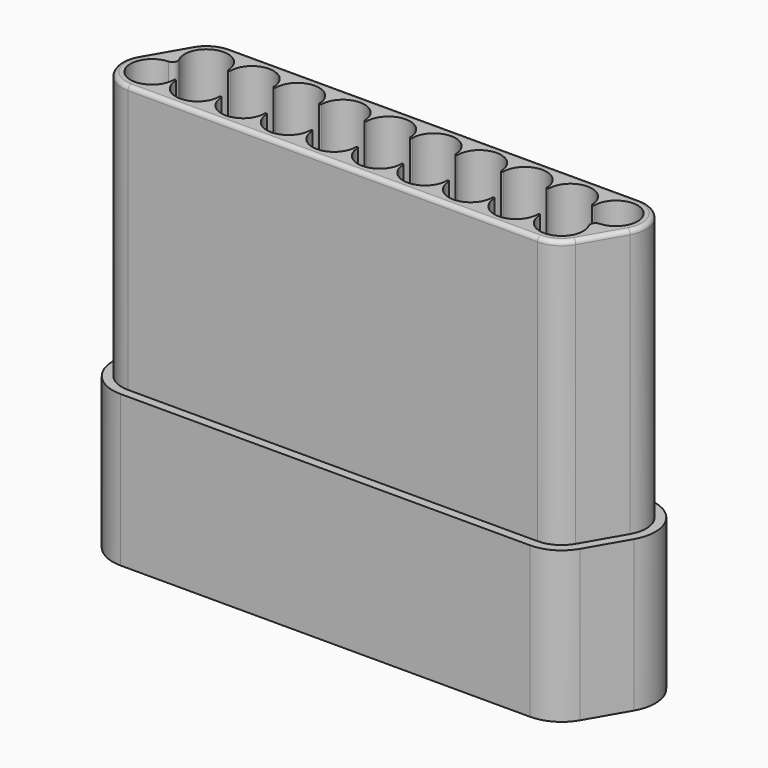
from build123d import *

# Parameters (mm, degrees)
F1_DEPTH = 75
F2_DEPTH = 25
F3_DEPTH = 3.2
F4_R     = 0.8


# Not quite as in the source:
# - a feature names something its author has since deleted; it is built from what else it names


with BuildPart() as f1:
    # F0 (on Top) → F1 (new body)
    with BuildSketch(Plane.XY):
        with BuildLine():
            Line((-0.6430435314, 10.1862159322), (-4.8930435314, 2.825))
            ThreePointArc((-4.8930435314, 2.825), (-4.8930435314, -2.825), (0, -5.65))
            Line((0, -5.65), (76.5, -5.65))
            ThreePointArc((76.5, -5.65), (79.325, -4.8930435314), (81.3930435314, -2.825))
            Line((81.3930435314, -2.825), (85.6430435314, 4.5362159322))
            ThreePointArc((85.6430435314, 4.5362159322), (85.6430435314, 10.1862159322), (80.75, 13.0112159322))
            Line((80.75, 13.0112159322), (4.25, 13.0112159322))
            ThreePointArc((4.25, 13.0112159322), (1.425, 12.2542594635), (-0.6430435314, 10.1862159322))
        make_face()
        with BuildLine():
            ThreePointArc((4.45, 0), (4.25, -0.2), (4.05, 0))
            ThreePointArc((4.05, 0), (-2.7957165477, -2.9302677326), (-0.1902315974, 4.0455298713))
            ThreePointArc((-0.1902315974, 4.0455298713), (0.6288230416, 4.5444261358), (0.651352561, 5.5031963925))
            ThreePointArc((0.651352561, 5.5031963925), (3.2939723142, 11.2967605024), (8.3, 7.3612159322))
            ThreePointArc((8.3, 7.3612159322), (8.5, 7.5612159322), (8.7, 7.3612159322))
            ThreePointArc((8.7, 7.3612159322), (12.75, 11.4112159322), (16.8, 7.3612159322))
            ThreePointArc((16.8, 7.3612159322), (17, 7.5612159322), (17.2, 7.3612159322))
            ThreePointArc((17.2, 7.3612159322), (21.25, 11.4112159322), (25.3, 7.3612159322))
            ThreePointArc((25.3, 7.3612159322), (25.5, 7.5612159322), (25.7, 7.3612159322))
            ThreePointArc((25.7, 7.3612159322), (29.75, 11.4112159322), (33.8, 7.3612159322))
            ThreePointArc((33.8, 7.3612159322), (34, 7.5612159322), (34.2, 7.3612159322))
            ThreePointArc((34.2, 7.3612159322), (38.25, 11.4112159322), (42.3, 7.3612159322))
            ThreePointArc((42.3, 7.3612159322), (42.5, 7.5612159322), (42.7, 7.3612159322))
            ThreePointArc((42.7, 7.3612159322), (46.75, 11.4112159322), (50.8, 7.3612159322))
            ThreePointArc((50.8, 7.3612159322), (51, 7.5612159322), (51.2, 7.3612159322))
            ThreePointArc((51.2, 7.3612159322), (55.25, 11.4112159322), (59.3, 7.3612159322))
            ThreePointArc((59.3, 7.3612159322), (59.5, 7.5612159322), (59.7, 7.3612159322))
            ThreePointArc((59.7, 7.3612159322), (63.75, 11.4112159322), (67.8, 7.3612159322))
            ThreePointArc((67.8, 7.3612159322), (68, 7.5612159322), (68.2, 7.3612159322))
            ThreePointArc((68.2, 7.3612159322), (72.25, 11.4112159322), (76.3, 7.3612159322))
            ThreePointArc((76.3, 7.3612159322), (76.5, 7.5612159322), (76.7, 7.3612159322))
            ThreePointArc((76.7, 7.3612159322), (80.75, 11.4112159322), (84.8, 7.3612159322))
            ThreePointArc((84.8, 7.3612159322), (83.6802677326, 4.5654993844), (80.9402315974, 3.3156860609))
            ThreePointArc((80.9402315974, 3.3156860609), (80.1211769584, 2.8167897964), (80.098647439, 1.8580195397))
            ThreePointArc((80.098647439, 1.8580195397), (80.4355445702, 0.9560276858), (80.55, 0))
            ThreePointArc((80.55, 0), (76.5, -4.05), (72.45, 0))
            ThreePointArc((72.45, 0), (72.25, -0.2), (72.05, 0))
            ThreePointArc((72.05, 0), (68, -4.05), (63.95, 0))
            ThreePointArc((63.95, 0), (63.75, -0.2), (63.55, 0))
            ThreePointArc((63.55, 0), (59.5, -4.05), (55.45, 0))
            ThreePointArc((55.45, 0), (55.25, -0.2), (55.05, 0))
            ThreePointArc((55.05, 0), (51, -4.05), (46.95, 0))
            ThreePointArc((46.95, 0), (46.75, -0.2), (46.55, 0))
            ThreePointArc((46.55, 0), (42.5, -4.05), (38.45, 0))
            ThreePointArc((38.45, 0), (38.25, -0.2), (38.05, 0))
            ThreePointArc((38.05, 0), (34, -4.05), (29.95, 0))
            ThreePointArc((29.95, 0), (29.75, -0.2), (29.55, 0))
            ThreePointArc((29.55, 0), (25.5, -4.05), (21.45, 0))
            ThreePointArc((21.45, 0), (21.25, -0.2), (21.05, 0))
            ThreePointArc((21.05, 0), (17, -4.05), (12.95, 0))
            ThreePointArc((12.95, 0), (12.75, -0.2), (12.55, 0))
            ThreePointArc((12.55, 0), (8.5, -4.05), (4.45, 0))
        make_face(mode=Mode.SUBTRACT)
        with BuildLine():
            ThreePointArc((4.45, 0), (4.25, 0.2), (4.05, 0))
            ThreePointArc((4.05, 0), (4.25, -0.2), (4.45, 0))
        make_face()
        with BuildLine():
            ThreePointArc((8.7, 7.3612159322), (8.5, 7.5612159322), (8.3, 7.3612159322))
            ThreePointArc((8.3, 7.3612159322), (8.5, 7.1612159322), (8.7, 7.3612159322))
        make_face()
        with BuildLine():
            ThreePointArc((12.95, 0), (12.75, 0.2), (12.55, 0))
            ThreePointArc((12.55, 0), (12.75, -0.2), (12.95, 0))
        make_face()
        with BuildLine():
            ThreePointArc((17.2, 7.3612159322), (17, 7.5612159322), (16.8, 7.3612159322))
            ThreePointArc((16.8, 7.3612159322), (17, 7.1612159322), (17.2, 7.3612159322))
        make_face()
        with BuildLine():
            ThreePointArc((21.45, 0), (21.25, 0.2), (21.05, 0))
            ThreePointArc((21.05, 0), (21.25, -0.2), (21.45, 0))
        make_face()
        with BuildLine():
            ThreePointArc((25.7, 7.3612159322), (25.5, 7.5612159322), (25.3, 7.3612159322))
            ThreePointArc((25.3, 7.3612159322), (25.5, 7.1612159322), (25.7, 7.3612159322))
        make_face()
        with BuildLine():
            ThreePointArc((29.95, 0), (29.75, 0.2), (29.55, 0))
            ThreePointArc((29.55, 0), (29.75, -0.2), (29.95, 0))
        make_face()
        with BuildLine():
            ThreePointArc((34.2, 7.3612159322), (34, 7.5612159322), (33.8, 7.3612159322))
            ThreePointArc((33.8, 7.3612159322), (34, 7.1612159322), (34.2, 7.3612159322))
        make_face()
        with BuildLine():
            ThreePointArc((38.45, 0), (38.25, 0.2), (38.05, 0))
            ThreePointArc((38.05, 0), (38.25, -0.2), (38.45, 0))
        make_face()
        with BuildLine():
            ThreePointArc((42.7, 7.3612159322), (42.5, 7.5612159322), (42.3, 7.3612159322))
            ThreePointArc((42.3, 7.3612159322), (42.5, 7.1612159322), (42.7, 7.3612159322))
        make_face()
        with BuildLine():
            ThreePointArc((46.95, 0), (46.75, 0.2), (46.55, 0))
            ThreePointArc((46.55, 0), (46.75, -0.2), (46.95, 0))
        make_face()
        with BuildLine():
            ThreePointArc((51.2, 7.3612159322), (51, 7.5612159322), (50.8, 7.3612159322))
            ThreePointArc((50.8, 7.3612159322), (51, 7.1612159322), (51.2, 7.3612159322))
        make_face()
        with BuildLine():
            ThreePointArc((55.45, 0), (55.25, 0.2), (55.05, 0))
            ThreePointArc((55.05, 0), (55.25, -0.2), (55.45, 0))
        make_face()
        with BuildLine():
            ThreePointArc((59.7, 7.3612159322), (59.5, 7.5612159322), (59.3, 7.3612159322))
            ThreePointArc((59.3, 7.3612159322), (59.5, 7.1612159322), (59.7, 7.3612159322))
        make_face()
        with BuildLine():
            ThreePointArc((63.95, 0), (63.75, 0.2), (63.55, 0))
            ThreePointArc((63.55, 0), (63.75, -0.2), (63.95, 0))
        make_face()
        with BuildLine():
            ThreePointArc((68.2, 7.3612159322), (68, 7.5612159322), (67.8, 7.3612159322))
            ThreePointArc((67.8, 7.3612159322), (68, 7.1612159322), (68.2, 7.3612159322))
        make_face()
        with BuildLine():
            ThreePointArc((72.45, 0), (72.25, 0.2), (72.05, 0))
            ThreePointArc((72.05, 0), (72.25, -0.2), (72.45, 0))
        make_face()
        with BuildLine():
            ThreePointArc((76.7, 7.3612159322), (76.5, 7.5612159322), (76.3, 7.3612159322))
            ThreePointArc((76.3, 7.3612159322), (76.5, 7.1612159322), (76.7, 7.3612159322))
        make_face()
    extrude(amount=F1_DEPTH)

    # F0 (on Top) → F2 (join)
    with BuildSketch(Plane.XY):
        with BuildLine():
            Line((-2.1152867178, 11.0362159322), (-6.3652867178, 3.675))
            ThreePointArc((-6.3652867178, 3.675), (-6.3652867178, -3.675), (0, -7.35))
            Line((0, -7.35), (76.5, -7.35))
            ThreePointArc((76.5, -7.35), (80.175, -6.3652867178), (82.8652867178, -3.675))
            Line((82.8652867178, -3.675), (87.1152867178, 3.6862159322))
            ThreePointArc((87.1152867178, 3.6862159322), (87.1152867178, 11.0362159322), (80.75, 14.7112159322))
            Line((80.75, 14.7112159322), (4.25, 14.7112159322))
            ThreePointArc((4.25, 14.7112159322), (0.575, 13.72650265), (-2.1152867178, 11.0362159322))
        make_face()
        with BuildLine():
            ThreePointArc((0, -5.65), (-4.8930435314, -2.825), (-4.8930435314, 2.825))
            Line((-4.8930435314, 2.825), (-0.6430435314, 10.1862159322))
            ThreePointArc((-0.6430435314, 10.1862159322), (1.425, 12.2542594635), (4.25, 13.0112159322))
            Line((4.25, 13.0112159322), (80.75, 13.0112159322))
            ThreePointArc((80.75, 13.0112159322), (85.6430435314, 10.1862159322), (85.6430435314, 4.5362159322))
            Line((85.6430435314, 4.5362159322), (81.3930435314, -2.825))
            ThreePointArc((81.3930435314, -2.825), (79.325, -4.8930435314), (76.5, -5.65))
            Line((76.5, -5.65), (0, -5.65))
        make_face(mode=Mode.SUBTRACT)
    extrude(amount=F2_DEPTH)

    # F0 (on Top) → F3 (join)
    with BuildSketch(Plane.XY):
        with BuildLine():
            Line((-2.1152867178, 11.0362159322), (-6.3652867178, 3.675))
            ThreePointArc((-6.3652867178, 3.675), (-6.3652867178, -3.675), (0, -7.35))
            Line((0, -7.35), (76.5, -7.35))
            ThreePointArc((76.5, -7.35), (80.175, -6.3652867178), (82.8652867178, -3.675))
            Line((82.8652867178, -3.675), (87.1152867178, 3.6862159322))
            ThreePointArc((87.1152867178, 3.6862159322), (87.1152867178, 11.0362159322), (80.75, 14.7112159322))
            Line((80.75, 14.7112159322), (4.25, 14.7112159322))
            ThreePointArc((4.25, 14.7112159322), (0.575, 13.72650265), (-2.1152867178, 11.0362159322))
        make_face()
        with BuildLine():
            ThreePointArc((0, -5.65), (-4.8930435314, -2.825), (-4.8930435314, 2.825))
            Line((-4.8930435314, 2.825), (-0.6430435314, 10.1862159322))
            ThreePointArc((-0.6430435314, 10.1862159322), (1.425, 12.2542594635), (4.25, 13.0112159322))
            Line((4.25, 13.0112159322), (80.75, 13.0112159322))
            ThreePointArc((80.75, 13.0112159322), (85.6430435314, 10.1862159322), (85.6430435314, 4.5362159322))
            Line((85.6430435314, 4.5362159322), (81.3930435314, -2.825))
            ThreePointArc((81.3930435314, -2.825), (79.325, -4.8930435314), (76.5, -5.65))
            Line((76.5, -5.65), (0, -5.65))
        make_face(mode=Mode.SUBTRACT)
        with BuildLine():
            Line((-0.6430435314, 10.1862159322), (-4.8930435314, 2.825))
            ThreePointArc((-4.8930435314, 2.825), (-4.8930435314, -2.825), (0, -5.65))
            Line((0, -5.65), (76.5, -5.65))
            ThreePointArc((76.5, -5.65), (79.325, -4.8930435314), (81.3930435314, -2.825))
            Line((81.3930435314, -2.825), (85.6430435314, 4.5362159322))
            ThreePointArc((85.6430435314, 4.5362159322), (85.6430435314, 10.1862159322), (80.75, 13.0112159322))
            Line((80.75, 13.0112159322), (4.25, 13.0112159322))
            ThreePointArc((4.25, 13.0112159322), (1.425, 12.2542594635), (-0.6430435314, 10.1862159322))
        make_face()
        with BuildLine():
            ThreePointArc((4.45, 0), (4.25, -0.2), (4.05, 0))
            ThreePointArc((4.05, 0), (-2.7957165477, -2.9302677326), (-0.1902315974, 4.0455298713))
            ThreePointArc((-0.1902315974, 4.0455298713), (0.6288230416, 4.5444261358), (0.651352561, 5.5031963925))
            ThreePointArc((0.651352561, 5.5031963925), (3.2939723142, 11.2967605024), (8.3, 7.3612159322))
            ThreePointArc((8.3, 7.3612159322), (8.5, 7.5612159322), (8.7, 7.3612159322))
            ThreePointArc((8.7, 7.3612159322), (12.75, 11.4112159322), (16.8, 7.3612159322))
            ThreePointArc((16.8, 7.3612159322), (17, 7.5612159322), (17.2, 7.3612159322))
            ThreePointArc((17.2, 7.3612159322), (21.25, 11.4112159322), (25.3, 7.3612159322))
            ThreePointArc((25.3, 7.3612159322), (25.5, 7.5612159322), (25.7, 7.3612159322))
            ThreePointArc((25.7, 7.3612159322), (29.75, 11.4112159322), (33.8, 7.3612159322))
            ThreePointArc((33.8, 7.3612159322), (34, 7.5612159322), (34.2, 7.3612159322))
            ThreePointArc((34.2, 7.3612159322), (38.25, 11.4112159322), (42.3, 7.3612159322))
            ThreePointArc((42.3, 7.3612159322), (42.5, 7.5612159322), (42.7, 7.3612159322))
            ThreePointArc((42.7, 7.3612159322), (46.75, 11.4112159322), (50.8, 7.3612159322))
            ThreePointArc((50.8, 7.3612159322), (51, 7.5612159322), (51.2, 7.3612159322))
            ThreePointArc((51.2, 7.3612159322), (55.25, 11.4112159322), (59.3, 7.3612159322))
            ThreePointArc((59.3, 7.3612159322), (59.5, 7.5612159322), (59.7, 7.3612159322))
            ThreePointArc((59.7, 7.3612159322), (63.75, 11.4112159322), (67.8, 7.3612159322))
            ThreePointArc((67.8, 7.3612159322), (68, 7.5612159322), (68.2, 7.3612159322))
            ThreePointArc((68.2, 7.3612159322), (72.25, 11.4112159322), (76.3, 7.3612159322))
            ThreePointArc((76.3, 7.3612159322), (76.5, 7.5612159322), (76.7, 7.3612159322))
            ThreePointArc((76.7, 7.3612159322), (80.75, 11.4112159322), (84.8, 7.3612159322))
            ThreePointArc((84.8, 7.3612159322), (83.6802677326, 4.5654993844), (80.9402315974, 3.3156860609))
            ThreePointArc((80.9402315974, 3.3156860609), (80.1211769584, 2.8167897964), (80.098647439, 1.8580195397))
            ThreePointArc((80.098647439, 1.8580195397), (80.4355445702, 0.9560276858), (80.55, 0))
            ThreePointArc((80.55, 0), (76.5, -4.05), (72.45, 0))
            ThreePointArc((72.45, 0), (72.25, -0.2), (72.05, 0))
            ThreePointArc((72.05, 0), (68, -4.05), (63.95, 0))
            ThreePointArc((63.95, 0), (63.75, -0.2), (63.55, 0))
            ThreePointArc((63.55, 0), (59.5, -4.05), (55.45, 0))
            ThreePointArc((55.45, 0), (55.25, -0.2), (55.05, 0))
            ThreePointArc((55.05, 0), (51, -4.05), (46.95, 0))
            ThreePointArc((46.95, 0), (46.75, -0.2), (46.55, 0))
            ThreePointArc((46.55, 0), (42.5, -4.05), (38.45, 0))
            ThreePointArc((38.45, 0), (38.25, -0.2), (38.05, 0))
            ThreePointArc((38.05, 0), (34, -4.05), (29.95, 0))
            ThreePointArc((29.95, 0), (29.75, -0.2), (29.55, 0))
            ThreePointArc((29.55, 0), (25.5, -4.05), (21.45, 0))
            ThreePointArc((21.45, 0), (21.25, -0.2), (21.05, 0))
            ThreePointArc((21.05, 0), (17, -4.05), (12.95, 0))
            ThreePointArc((12.95, 0), (12.75, -0.2), (12.55, 0))
            ThreePointArc((12.55, 0), (8.5, -4.05), (4.45, 0))
        make_face(mode=Mode.SUBTRACT)
        with BuildLine():
            ThreePointArc((-0.1902315974, 4.0455298713), (2.7957165477, 2.9302677326), (4.05, 0))
            ThreePointArc((4.05, 0), (4.25, 0.2), (4.45, 0))
            ThreePointArc((4.45, 0), (8.5, 4.05), (12.55, 0))
            ThreePointArc((12.55, 0), (12.75, 0.2), (12.95, 0))
            ThreePointArc((12.95, 0), (17, 4.05), (21.05, 0))
            ThreePointArc((21.05, 0), (21.25, 0.2), (21.45, 0))
            ThreePointArc((21.45, 0), (25.5, 4.05), (29.55, 0))
            ThreePointArc((29.55, 0), (29.75, 0.2), (29.95, 0))
            ThreePointArc((29.95, 0), (34, 4.05), (38.05, 0))
            ThreePointArc((38.05, 0), (38.25, 0.2), (38.45, 0))
            ThreePointArc((38.45, 0), (42.5, 4.05), (46.55, 0))
            ThreePointArc((46.55, 0), (46.75, 0.2), (46.95, 0))
            ThreePointArc((46.95, 0), (51, 4.05), (55.05, 0))
            ThreePointArc((55.05, 0), (55.25, 0.2), (55.45, 0))
            ThreePointArc((55.45, 0), (59.5, 4.05), (63.55, 0))
            ThreePointArc((63.55, 0), (63.75, 0.2), (63.95, 0))
            ThreePointArc((63.95, 0), (68, 4.05), (72.05, 0))
            ThreePointArc((72.05, 0), (72.25, 0.2), (72.45, 0))
            ThreePointArc((72.45, 0), (75.5439723142, 3.9355445702), (80.098647439, 1.8580195397))
            ThreePointArc((80.098647439, 1.8580195397), (80.1211769584, 2.8167897964), (80.9402315974, 3.3156860609))
            ThreePointArc((80.9402315974, 3.3156860609), (77.9542834523, 4.4309481996), (76.7, 7.3612159322))
            ThreePointArc((76.7, 7.3612159322), (76.5, 7.1612159322), (76.3, 7.3612159322))
            ThreePointArc((76.3, 7.3612159322), (72.25, 3.3112159322), (68.2, 7.3612159322))
            ThreePointArc((68.2, 7.3612159322), (68, 7.1612159322), (67.8, 7.3612159322))
            ThreePointArc((67.8, 7.3612159322), (63.75, 3.3112159322), (59.7, 7.3612159322))
            ThreePointArc((59.7, 7.3612159322), (59.5, 7.1612159322), (59.3, 7.3612159322))
            ThreePointArc((59.3, 7.3612159322), (55.25, 3.3112159322), (51.2, 7.3612159322))
            ThreePointArc((51.2, 7.3612159322), (51, 7.1612159322), (50.8, 7.3612159322))
            ThreePointArc((50.8, 7.3612159322), (46.75, 3.3112159322), (42.7, 7.3612159322))
            ThreePointArc((42.7, 7.3612159322), (42.5, 7.1612159322), (42.3, 7.3612159322))
            ThreePointArc((42.3, 7.3612159322), (38.25, 3.3112159322), (34.2, 7.3612159322))
            ThreePointArc((34.2, 7.3612159322), (34, 7.1612159322), (33.8, 7.3612159322))
            ThreePointArc((33.8, 7.3612159322), (29.75, 3.3112159322), (25.7, 7.3612159322))
            ThreePointArc((25.7, 7.3612159322), (25.5, 7.1612159322), (25.3, 7.3612159322))
            ThreePointArc((25.3, 7.3612159322), (21.25, 3.3112159322), (17.2, 7.3612159322))
            ThreePointArc((17.2, 7.3612159322), (17, 7.1612159322), (16.8, 7.3612159322))
            ThreePointArc((16.8, 7.3612159322), (12.75, 3.3112159322), (8.7, 7.3612159322))
            ThreePointArc((8.7, 7.3612159322), (8.5, 7.1612159322), (8.3, 7.3612159322))
            ThreePointArc((8.3, 7.3612159322), (5.2060276858, 3.425671362), (0.651352561, 5.5031963925))
            ThreePointArc((0.651352561, 5.5031963925), (0.6288230416, 4.5444261358), (-0.1902315974, 4.0455298713))
        make_face()
        with BuildLine():
            ThreePointArc((-0.1902315974, 4.0455298713), (-2.7957165477, -2.9302677326), (4.05, 0))
            ThreePointArc((4.05, 0), (2.7957165477, 2.9302677326), (-0.1902315974, 4.0455298713))
        make_face()
        with BuildLine():
            ThreePointArc((12.55, 0), (8.5, 4.05), (4.45, 0))
            ThreePointArc((4.45, 0), (8.5, -4.05), (12.55, 0))
        make_face()
        with BuildLine():
            ThreePointArc((8.3, 7.3612159322), (3.2939723142, 11.2967605024), (0.651352561, 5.5031963925))
            ThreePointArc((0.651352561, 5.5031963925), (5.2060276858, 3.425671362), (8.3, 7.3612159322))
        make_face()
        with BuildLine():
            ThreePointArc((21.05, 0), (17, 4.05), (12.95, 0))
            ThreePointArc((12.95, 0), (17, -4.05), (21.05, 0))
        make_face()
        with BuildLine():
            ThreePointArc((16.8, 7.3612159322), (12.75, 11.4112159322), (8.7, 7.3612159322))
            ThreePointArc((8.7, 7.3612159322), (12.75, 3.3112159322), (16.8, 7.3612159322))
        make_face()
        with BuildLine():
            ThreePointArc((29.55, 0), (25.5, 4.05), (21.45, 0))
            ThreePointArc((21.45, 0), (25.5, -4.05), (29.55, 0))
        make_face()
        with BuildLine():
            ThreePointArc((25.3, 7.3612159322), (21.25, 11.4112159322), (17.2, 7.3612159322))
            ThreePointArc((17.2, 7.3612159322), (21.25, 3.3112159322), (25.3, 7.3612159322))
        make_face()
        with BuildLine():
            ThreePointArc((38.05, 0), (34, 4.05), (29.95, 0))
            ThreePointArc((29.95, 0), (34, -4.05), (38.05, 0))
        make_face()
        with BuildLine():
            ThreePointArc((33.8, 7.3612159322), (29.75, 11.4112159322), (25.7, 7.3612159322))
            ThreePointArc((25.7, 7.3612159322), (29.75, 3.3112159322), (33.8, 7.3612159322))
        make_face()
        with BuildLine():
            ThreePointArc((46.55, 0), (42.5, 4.05), (38.45, 0))
            ThreePointArc((38.45, 0), (42.5, -4.05), (46.55, 0))
        make_face()
        with BuildLine():
            ThreePointArc((42.3, 7.3612159322), (38.25, 11.4112159322), (34.2, 7.3612159322))
            ThreePointArc((34.2, 7.3612159322), (38.25, 3.3112159322), (42.3, 7.3612159322))
        make_face()
        with BuildLine():
            ThreePointArc((55.05, 0), (51, 4.05), (46.95, 0))
            ThreePointArc((46.95, 0), (51, -4.05), (55.05, 0))
        make_face()
        with BuildLine():
            ThreePointArc((50.8, 7.3612159322), (46.75, 11.4112159322), (42.7, 7.3612159322))
            ThreePointArc((42.7, 7.3612159322), (46.75, 3.3112159322), (50.8, 7.3612159322))
        make_face()
        with BuildLine():
            ThreePointArc((63.55, 0), (59.5, 4.05), (55.45, 0))
            ThreePointArc((55.45, 0), (59.5, -4.05), (63.55, 0))
        make_face()
        with BuildLine():
            ThreePointArc((59.3, 7.3612159322), (55.25, 11.4112159322), (51.2, 7.3612159322))
            ThreePointArc((51.2, 7.3612159322), (55.25, 3.3112159322), (59.3, 7.3612159322))
        make_face()
        with BuildLine():
            ThreePointArc((72.05, 0), (68, 4.05), (63.95, 0))
            ThreePointArc((63.95, 0), (68, -4.05), (72.05, 0))
        make_face()
        with BuildLine():
            ThreePointArc((67.8, 7.3612159322), (63.75, 11.4112159322), (59.7, 7.3612159322))
            ThreePointArc((59.7, 7.3612159322), (63.75, 3.3112159322), (67.8, 7.3612159322))
        make_face()
        with BuildLine():
            ThreePointArc((80.098647439, 1.8580195397), (75.5439723142, 3.9355445702), (72.45, 0))
            ThreePointArc((72.45, 0), (76.5, -4.05), (80.55, 0))
            ThreePointArc((80.55, 0), (80.4355445702, 0.9560276858), (80.098647439, 1.8580195397))
        make_face()
        with BuildLine():
            ThreePointArc((76.3, 7.3612159322), (72.25, 11.4112159322), (68.2, 7.3612159322))
            ThreePointArc((68.2, 7.3612159322), (72.25, 3.3112159322), (76.3, 7.3612159322))
        make_face()
        with BuildLine():
            ThreePointArc((76.7, 7.3612159322), (77.9542834523, 4.4309481996), (80.9402315974, 3.3156860609))
            ThreePointArc((80.9402315974, 3.3156860609), (83.6802677326, 4.5654993844), (84.8, 7.3612159322))
            ThreePointArc((84.8, 7.3612159322), (80.75, 11.4112159322), (76.7, 7.3612159322))
        make_face()
        with BuildLine():
            ThreePointArc((4.45, 0), (4.25, 0.2), (4.05, 0))
            ThreePointArc((4.05, 0), (4.25, -0.2), (4.45, 0))
        make_face()
        with BuildLine():
            ThreePointArc((12.95, 0), (12.75, 0.2), (12.55, 0))
            ThreePointArc((12.55, 0), (12.75, -0.2), (12.95, 0))
        make_face()
        with BuildLine():
            ThreePointArc((8.7, 7.3612159322), (8.5, 7.5612159322), (8.3, 7.3612159322))
            ThreePointArc((8.3, 7.3612159322), (8.5, 7.1612159322), (8.7, 7.3612159322))
        make_face()
        with BuildLine():
            ThreePointArc((21.45, 0), (21.25, 0.2), (21.05, 0))
            ThreePointArc((21.05, 0), (21.25, -0.2), (21.45, 0))
        make_face()
        with BuildLine():
            ThreePointArc((17.2, 7.3612159322), (17, 7.5612159322), (16.8, 7.3612159322))
            ThreePointArc((16.8, 7.3612159322), (17, 7.1612159322), (17.2, 7.3612159322))
        make_face()
        with BuildLine():
            ThreePointArc((29.95, 0), (29.75, 0.2), (29.55, 0))
            ThreePointArc((29.55, 0), (29.75, -0.2), (29.95, 0))
        make_face()
        with BuildLine():
            ThreePointArc((25.7, 7.3612159322), (25.5, 7.5612159322), (25.3, 7.3612159322))
            ThreePointArc((25.3, 7.3612159322), (25.5, 7.1612159322), (25.7, 7.3612159322))
        make_face()
        with BuildLine():
            ThreePointArc((38.45, 0), (38.25, 0.2), (38.05, 0))
            ThreePointArc((38.05, 0), (38.25, -0.2), (38.45, 0))
        make_face()
        with BuildLine():
            ThreePointArc((34.2, 7.3612159322), (34, 7.5612159322), (33.8, 7.3612159322))
            ThreePointArc((33.8, 7.3612159322), (34, 7.1612159322), (34.2, 7.3612159322))
        make_face()
        with BuildLine():
            ThreePointArc((46.95, 0), (46.75, 0.2), (46.55, 0))
            ThreePointArc((46.55, 0), (46.75, -0.2), (46.95, 0))
        make_face()
        with BuildLine():
            ThreePointArc((42.7, 7.3612159322), (42.5, 7.5612159322), (42.3, 7.3612159322))
            ThreePointArc((42.3, 7.3612159322), (42.5, 7.1612159322), (42.7, 7.3612159322))
        make_face()
        with BuildLine():
            ThreePointArc((55.45, 0), (55.25, 0.2), (55.05, 0))
            ThreePointArc((55.05, 0), (55.25, -0.2), (55.45, 0))
        make_face()
        with BuildLine():
            ThreePointArc((51.2, 7.3612159322), (51, 7.5612159322), (50.8, 7.3612159322))
            ThreePointArc((50.8, 7.3612159322), (51, 7.1612159322), (51.2, 7.3612159322))
        make_face()
        with BuildLine():
            ThreePointArc((63.95, 0), (63.75, 0.2), (63.55, 0))
            ThreePointArc((63.55, 0), (63.75, -0.2), (63.95, 0))
        make_face()
        with BuildLine():
            ThreePointArc((59.7, 7.3612159322), (59.5, 7.5612159322), (59.3, 7.3612159322))
            ThreePointArc((59.3, 7.3612159322), (59.5, 7.1612159322), (59.7, 7.3612159322))
        make_face()
        with BuildLine():
            ThreePointArc((72.45, 0), (72.25, 0.2), (72.05, 0))
            ThreePointArc((72.05, 0), (72.25, -0.2), (72.45, 0))
        make_face()
        with BuildLine():
            ThreePointArc((68.2, 7.3612159322), (68, 7.5612159322), (67.8, 7.3612159322))
            ThreePointArc((67.8, 7.3612159322), (68, 7.1612159322), (68.2, 7.3612159322))
        make_face()
        with BuildLine():
            ThreePointArc((76.7, 7.3612159322), (76.5, 7.5612159322), (76.3, 7.3612159322))
            ThreePointArc((76.3, 7.3612159322), (76.5, 7.1612159322), (76.7, 7.3612159322))
        make_face()
    extrude(amount=-F3_DEPTH)

    # F4
    f4_edges = [f1.edges().sort_by_distance(p)[0] for p in [
        (38.25, -5.65, 75),
        (85.643044, 10.186216, 75),
        (83.518044, 0.855608, 75),
        (79.325, -4.893044, 75),
        (-4.893044, -2.825, 75),
        (-2.768044, 6.505608, 75),
        (1.425, 12.254259, 75),
        (42.5, 13.011216, 75),
    ]]
    fillet(f4_edges, radius=F4_R)


solid = f1.part
